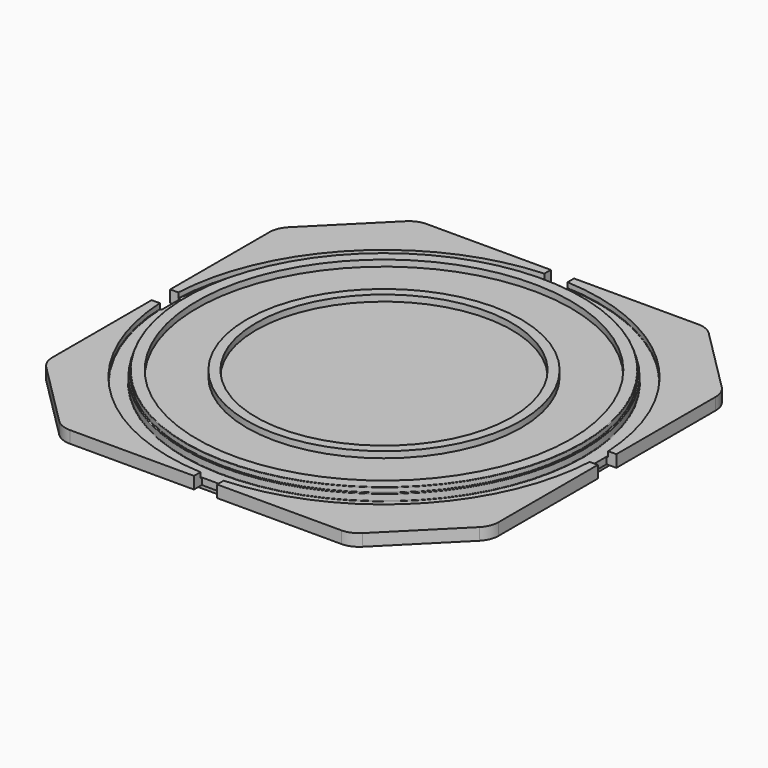
from build123d import *

# Parameters (mm, degrees)
F0_W            = 1000
F0_H            = 1000
F1_DEPTH        = 51
F2_SIZE         = 175
F3_R            = 50
F5_W            = 52
F5_H            = 100
F6_DEPTH        = 100
F6_COPIES_COUNT = 4
F7_R            = 410
F8_DEPTH        = 10
F9_W            = 1332.0814967155
F9_H            = 1389.9142146111
F10_DEPTH       = 10
F11_R           = 120
F12_R           = 700
F12_R_2         = 444
F13_DEPTH       = 11
F14_R           = 700
F14_R_2         = 447.5
F15_DEPTH       = 14
F16_R           = 482.5
F16_R_2         = 447.5
F17_DEPTH       = 26
F18_R           = 1
F19_R           = 419
F19_R_2         = 307.5
F20_DEPTH       = 14
F21_R           = 286.5
F22_DEPTH       = 14


# Not quite as in the source:
# - a pattern or mirror of a feature is missing from the dataset's text; its kind, count and spacing are read off the source's solid


with BuildPart() as f1:
    # F0 (on Top) → F1 (new body)
    with BuildSketch(Plane.XY):
        Rectangle(F0_W, F0_H)
    extrude(amount=F1_DEPTH)

    # F2
    f2_edges = [f1.edges().sort_by_distance(p)[0] for p in [
        (-500, -500, 25.5),
        (500, -500, 25.5),
        (500, 500, 25.5),
        (-500, 500, 25.5),
    ]]
    chamfer(f2_edges, length=F2_SIZE)

    # F3
    f3_edges = [f1.edges().sort_by_distance(p)[0] for p in [
        (-500, -325, 25.5),
        (-325, -500, 25.5),
        (325, -500, 25.5),
        (500, -325, 25.5),
        (-500, 325, 25.5),
        (500, 325, 25.5),
        (325, 500, 25.5),
        (-325, 500, 25.5),
    ]]
    fillet(f3_edges, radius=F3_R)

    # F5 (on face) → F6 (cut)
    with BuildSketch(Plane.XY.offset(51)):
        with Locations((0, 528)):
            Rectangle(F5_W, F5_H)
    f6 = extrude(amount=-F6_DEPTH, mode=Mode.SUBTRACT)

    # F6_copies: F6 ×4 about axis
    f6_copies_axis = Axis((0, 0, 0), (0, 0, 1))
    for i in range(1, F6_COPIES_COUNT):
        add(f6.rotate(f6_copies_axis, i * 360 / F6_COPIES_COUNT), mode=Mode.SUBTRACT)

    # F7 (on Top) → F8 (cut)
    with BuildSketch(Plane.XY):
        Circle(F7_R)
    extrude(amount=F8_DEPTH, mode=Mode.SUBTRACT)

    # F9 (on Top) → F10 (cut)
    with BuildSketch(Plane.XY):
        with Locations((-30.3454697132, 79.7554552555)):
            Rectangle(F9_W, F9_H)
        Polygon((473, 313.8162338159), (473, -313.8162338159), (313.8162338159, -473), (-313.8162338159, -473), (-473, -313.8162338159), (-473, 313.8162338159), (-313.8162338159, 473), (313.8162338159, 473), align=None, mode=Mode.SUBTRACT)
    extrude(amount=F10_DEPTH, mode=Mode.SUBTRACT)

    # F11
    f11_edges = [f1.edges().sort_by_distance(p)[0] for p in [
        (-313.816234, -473, 5),
        (-473, -313.816234, 5),
        (-473, 313.816234, 5),
        (-313.816234, 473, 5),
        (473, -313.816234, 5),
        (313.816234, -473, 5),
        (313.816234, 473, 5),
        (473, 313.816234, 5),
    ]]
    fillet(f11_edges, radius=F11_R)

    # F12 (on face) → F13 (cut)
    with BuildSketch(Plane.XY.offset(51)):
        Circle(F12_R)
        Circle(F12_R_2, mode=Mode.SUBTRACT)
    extrude(amount=-F13_DEPTH, mode=Mode.SUBTRACT)

    # F14 (on face) → F15 (cut)
    with BuildSketch(Plane.XY.offset(51)):
        Circle(F14_R)
        Circle(F14_R_2, mode=Mode.SUBTRACT)
    extrude(amount=-F15_DEPTH, mode=Mode.SUBTRACT)

    # F16 (on face) → F17 (cut)
    with BuildSketch(Plane.XY.offset(51)):
        Circle(F16_R)
        Circle(F16_R_2, mode=Mode.SUBTRACT)
    extrude(amount=-F17_DEPTH, mode=Mode.SUBTRACT)

    # F18
    f18_edges = [f1.edges().sort_by_distance(p)[0] for p in [
        (-341.179022, 341.179022, 25),
        (341.179022, 341.179022, 25),
        (341.179022, -341.179022, 25),
        (-341.179022, -341.179022, 25),
        (-447.5, 0, 25),
        (-444, 0, 40),
        (-447.5, 0, 40),
        (-444, 0, 51),
    ]]
    fillet(f18_edges, radius=F18_R)

    # F19 (on face) → F20 (cut)
    with BuildSketch(Plane.XY.offset(51)):
        Circle(F19_R)
        Circle(F19_R_2, mode=Mode.SUBTRACT)
    extrude(amount=-F20_DEPTH, mode=Mode.SUBTRACT)

    # F21 (on face) → F22 (cut)
    with BuildSketch(Plane.XY.offset(51)):
        Circle(F21_R)
    extrude(amount=-F22_DEPTH, mode=Mode.SUBTRACT)


solid = f1.part
